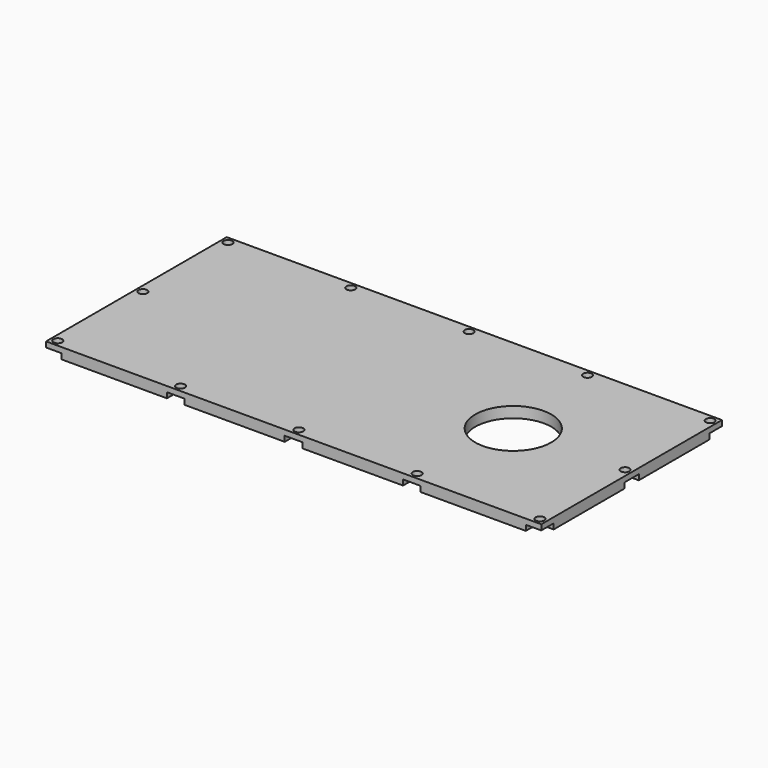
from build123d import *

# Parameters (mm, degrees)
F0_R     = 23.5
F0_R_2   = 17.5
F1_DEPTH = 5
F0_R_3   = 2
F2_DEPTH = 2.5


# Not quite as in the source:
# - a feature names something its author has since deleted; it is built from what else it names


with BuildPart() as f1:
    # F0 (on Top) → F1 (new body)
    with BuildSketch(Plane.XY):
        with BuildLine():
            Line((-58.3766478719, 52), (-106.8995, 52))
            Line((-106.8995, 52), (-106.8995, 49))
            ThreePointArc((-106.8995, 49), (-108.1076845276, 46.0831845276), (-111.0245, 44.875))
            Line((-111.0245, 44.875), (-114.0245, 44.875))
            Line((-114.0245, 44.875), (-114.0245, 4.125))
            Line((-114.0245, 4.125), (-111.0245, 4.125))
            ThreePointArc((-111.0245, 4.125), (-106.8995, 0), (-111.0245, -4.125))
            Line((-111.0245, -4.125), (-114.0245, -4.125))
            Line((-114.0245, -4.125), (-114.0245, -44.875))
            Line((-114.0245, -44.875), (-111.0245, -44.875))
            ThreePointArc((-111.0245, -44.875), (-108.1076845276, -46.0831845276), (-106.8995, -49))
            Line((-106.8995, -49), (-106.8995, -52))
            Line((-106.8995, -52), (-58.3766478719, -52))
            Line((-58.3766478719, -52), (-58.3766478719, -47.5903098648))
            ThreePointArc((-58.3766478719, -47.5903098648), (-53.7843001577, -44.9375624638), (-50.375, -49))
            Line((-50.375, -49), (-50.375, -52))
            Line((-50.375, -52), (-4.125, -52))
            Line((-4.125, -52), (-4.125, -49))
            ThreePointArc((-4.125, -49), (0, -44.875), (4.125, -49))
            Line((4.125, -49), (4.125, -52))
            Line((4.125, -52), (50.375, -52))
            Line((50.375, -52), (50.375, -49))
            ThreePointArc((50.375, -49), (53.7843001577, -44.9375624638), (58.3766478719, -47.5903098648))
            Line((58.3766478719, -47.5903098648), (58.3766478719, -52))
            Line((58.3766478719, -52), (106.8995, -52))
            Line((106.8995, -52), (106.8995, -49))
            ThreePointArc((106.8995, -49), (108.1076845276, -46.0831845276), (111.0245, -44.875))
            Line((111.0245, -44.875), (114.0245, -44.875))
            Line((114.0245, -44.875), (114.0245, -4.125))
            Line((114.0245, -4.125), (111.0245, -4.125))
            ThreePointArc((111.0245, -4.125), (106.8995, 0), (111.0245, 4.125))
            Line((111.0245, 4.125), (114.0245, 4.125))
            Line((114.0245, 4.125), (114.0245, 44.875))
            Line((114.0245, 44.875), (111.0245, 44.875))
            ThreePointArc((111.0245, 44.875), (108.1076845276, 46.0831845276), (106.8995, 49))
            Line((106.8995, 49), (106.8995, 52))
            Line((106.8995, 52), (58.3766478719, 52))
            Line((58.3766478719, 52), (58.3766478719, 47.5903098648))
            ThreePointArc((58.3766478719, 47.5903098648), (53.7843001577, 44.9375624638), (50.375, 49))
            Line((50.375, 49), (50.375, 52))
            Line((50.375, 52), (4.125, 52))
            Line((4.125, 52), (4.125, 49))
            ThreePointArc((4.125, 49), (0, 44.875), (-4.125, 49))
            Line((-4.125, 49), (-4.125, 52))
            Line((-4.125, 52), (-50.375, 52))
            Line((-50.375, 52), (-50.375, 49))
            ThreePointArc((-50.375, 49), (-53.7843001577, 44.9375624638), (-58.3766478719, 47.5903098648))
            Line((-58.3766478719, 47.5903098648), (-58.3766478719, 52))
        make_face()
        with Locations((59.5245, 0)):
            Circle(F0_R, mode=Mode.SUBTRACT)
        with Locations((59.5245, 0)):
            Circle(F0_R)
        with Locations((59.5245, 0)):
            Circle(F0_R_2, mode=Mode.SUBTRACT)
    extrude(amount=-F1_DEPTH)

    # F0 (on Top) → F2 (join)
    with BuildSketch(Plane.XY):
        with BuildLine():
            Line((-106.8995, 52), (-114.0245, 52))
            Line((-114.0245, 52), (-114.0245, 44.875))
            Line((-114.0245, 44.875), (-111.0245, 44.875))
            ThreePointArc((-111.0245, 44.875), (-108.1076845276, 46.0831845276), (-106.8995, 49))
            Line((-106.8995, 49), (-106.8995, 52))
        make_face()
        with Locations((-111.0245, 49)):
            Circle(F0_R_3, mode=Mode.SUBTRACT)
        with BuildLine():
            Line((-111.0245, 4.125), (-114.0245, 4.125))
            Line((-114.0245, 4.125), (-114.0245, -4.125))
            Line((-114.0245, -4.125), (-111.0245, -4.125))
            ThreePointArc((-111.0245, -4.125), (-106.8995, 0), (-111.0245, 4.125))
        make_face()
        with Locations((-111.0245, 0)):
            Circle(F0_R_3, mode=Mode.SUBTRACT)
        with BuildLine():
            Line((-111.0245, -44.875), (-114.0245, -44.875))
            Line((-114.0245, -44.875), (-114.0245, -52))
            Line((-114.0245, -52), (-106.8995, -52))
            Line((-106.8995, -52), (-106.8995, -49))
            ThreePointArc((-106.8995, -49), (-108.1076845276, -46.0831845276), (-111.0245, -44.875))
        make_face()
        with Locations((-111.0245, -49)):
            Circle(F0_R_3, mode=Mode.SUBTRACT)
        with BuildLine():
            Line((-58.3766478719, -47.5903098648), (-58.3766478719, -52))
            Line((-58.3766478719, -52), (-50.375, -52))
            Line((-50.375, -52), (-50.375, -49))
            ThreePointArc((-50.375, -49), (-53.7843001577, -44.9375624638), (-58.3766478719, -47.5903098648))
        make_face()
        with Locations((-54.5, -49)):
            Circle(F0_R_3, mode=Mode.SUBTRACT)
        with BuildLine():
            Line((-4.125, -49), (-4.125, -52))
            Line((-4.125, -52), (4.125, -52))
            Line((4.125, -52), (4.125, -49))
            ThreePointArc((4.125, -49), (0, -44.875), (-4.125, -49))
        make_face()
        with Locations((0, -49)):
            Circle(F0_R_3, mode=Mode.SUBTRACT)
        with BuildLine():
            Line((50.375, -49), (50.375, -52))
            Line((50.375, -52), (58.3766478719, -52))
            Line((58.3766478719, -52), (58.3766478719, -47.5903098648))
            ThreePointArc((58.3766478719, -47.5903098648), (53.7843001577, -44.9375624638), (50.375, -49))
        make_face()
        with Locations((54.5, -49)):
            Circle(F0_R_3, mode=Mode.SUBTRACT)
        with BuildLine():
            Line((114.0245, -52), (114.0245, -44.875))
            Line((114.0245, -44.875), (111.0245, -44.875))
            ThreePointArc((111.0245, -44.875), (108.1076845276, -46.0831845276), (106.8995, -49))
            Line((106.8995, -49), (106.8995, -52))
            Line((106.8995, -52), (114.0245, -52))
        make_face()
        with Locations((111.0245, -49)):
            Circle(F0_R_3, mode=Mode.SUBTRACT)
        with BuildLine():
            Line((114.0245, -4.125), (114.0245, 4.125))
            Line((114.0245, 4.125), (111.0245, 4.125))
            ThreePointArc((111.0245, 4.125), (106.8995, 0), (111.0245, -4.125))
            Line((111.0245, -4.125), (114.0245, -4.125))
        make_face()
        with Locations((111.0245, 0)):
            Circle(F0_R_3, mode=Mode.SUBTRACT)
        with BuildLine():
            Line((114.0245, 52), (106.8995, 52))
            Line((106.8995, 52), (106.8995, 49))
            ThreePointArc((106.8995, 49), (108.1076845276, 46.0831845276), (111.0245, 44.875))
            Line((111.0245, 44.875), (114.0245, 44.875))
            Line((114.0245, 44.875), (114.0245, 52))
        make_face()
        with Locations((111.0245, 49)):
            Circle(F0_R_3, mode=Mode.SUBTRACT)
        with BuildLine():
            Line((58.3766478719, 52), (50.375, 52))
            Line((50.375, 52), (50.375, 49))
            ThreePointArc((50.375, 49), (53.7843001577, 44.9375624638), (58.3766478719, 47.5903098648))
            Line((58.3766478719, 47.5903098648), (58.3766478719, 52))
        make_face()
        with Locations((54.5, 49)):
            Circle(F0_R_3, mode=Mode.SUBTRACT)
        with BuildLine():
            Line((4.125, 52), (-4.125, 52))
            Line((-4.125, 52), (-4.125, 49))
            ThreePointArc((-4.125, 49), (0, 44.875), (4.125, 49))
            Line((4.125, 49), (4.125, 52))
        make_face()
        with Locations((0, 49)):
            Circle(F0_R_3, mode=Mode.SUBTRACT)
        with BuildLine():
            Line((-50.375, 52), (-58.3766478719, 52))
            Line((-58.3766478719, 52), (-58.3766478719, 47.5903098648))
            ThreePointArc((-58.3766478719, 47.5903098648), (-53.7843001577, 44.9375624638), (-50.375, 49))
            Line((-50.375, 49), (-50.375, 52))
        make_face()
        with Locations((-54.5, 49)):
            Circle(F0_R_3, mode=Mode.SUBTRACT)
    extrude(amount=-F2_DEPTH)


solid = f1.part
